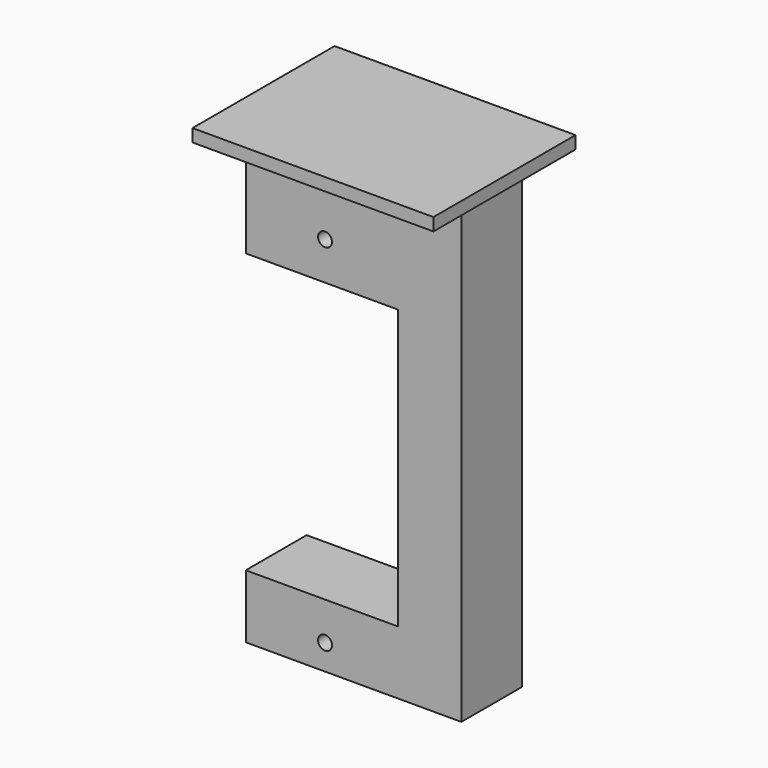
from build123d import *

# Parameters (mm, degrees)
F0_R     = 0.55
F1_DEPTH = 6
F2_DEPTH = 4
F3_W     = 19
F3_H     = 14
F3_W_2   = 17
F3_H_2   = 6
F4_DEPTH = 1


with BuildPart() as f1:
    # F0 (on Front) → F1 (new body)
    with BuildSketch(Plane.XZ):
        Polygon((0, 5), (0, 0), (12, 0), (12, -22), (0, -22), (0, -27), (12, -27), (17, -27), (17, 5), (12, 5), align=None)
        with Locations((6.25, -25)):
            Circle(F0_R, mode=Mode.SUBTRACT)
        with Locations((6.25, 3)):
            Circle(F0_R, mode=Mode.SUBTRACT)
    extrude(amount=F1_DEPTH)

    # F2 (add): a face of the model
    f2_faces = [f1.faces().sort_by_distance(p)[0] for p in [
        (8.5, -3, 5),
    ]]
    extrude(f2_faces, amount=F2_DEPTH)

    # F3 (on face) → F4 (join)
    with BuildSketch(Plane.XY.offset(9)):
        with Locations((8.5, -3)):
            Rectangle(F3_W, F3_H)
        with Locations((8.5, -3)):
            Rectangle(F3_W_2, F3_H_2, mode=Mode.SUBTRACT)
        with Locations((8.5, -3)):
            Rectangle(F3_W_2, F3_H_2)
    extrude(amount=F4_DEPTH)


solid = f1.part
